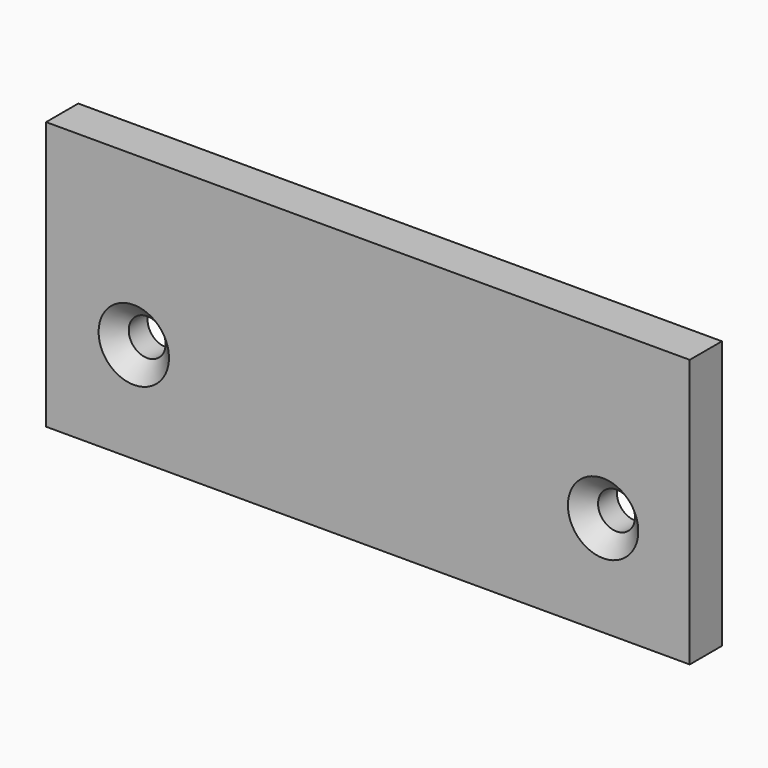
from build123d import *

# Parameters (mm, degrees)
F0_W           = 152.4
F0_H           = 63.5
F1_DEPTH       = 9.525
F2_R           = 4.365625
F3_DEPTH       = 25.4
F4_D           = 8.73125
F4_CSINK_D     = 16.66875
F4_CSINK_ANGLE = 90


# Not quite as in the source:
# - a length typed as a fraction of an inch, garbled in the dataset ("3 / 203.2 mm" for 3/8 in), is restored


with BuildPart() as f1:
    # F0 (on Front) → F1 (new body)
    with BuildSketch(Plane.XZ):
        with Locations((-2.7878060937, -27.0196995885)):
            Rectangle(F0_W, F0_H)
    extrude(amount=F1_DEPTH)

    # F2 (on face) → F3 (cut)
    with BuildSketch(Plane.XZ.offset(9.525)):
        with Locations((52.9022132752, -34.9571995885)):
            Circle(F2_R)
        with Locations((-58.2227867248, -34.9571995885)):
            Circle(F2_R)
    extrude(amount=-F3_DEPTH, mode=Mode.SUBTRACT)

    # F4 (through all)
    with Locations(Plane.XZ.offset(9.525)):
        with Locations((52.9022132752, -34.9571995885), (-58.2227867248, -34.9571995885)):
            CounterSinkHole(F4_D / 2, F4_CSINK_D / 2, counter_sink_angle=F4_CSINK_ANGLE)


solid = f1.part
